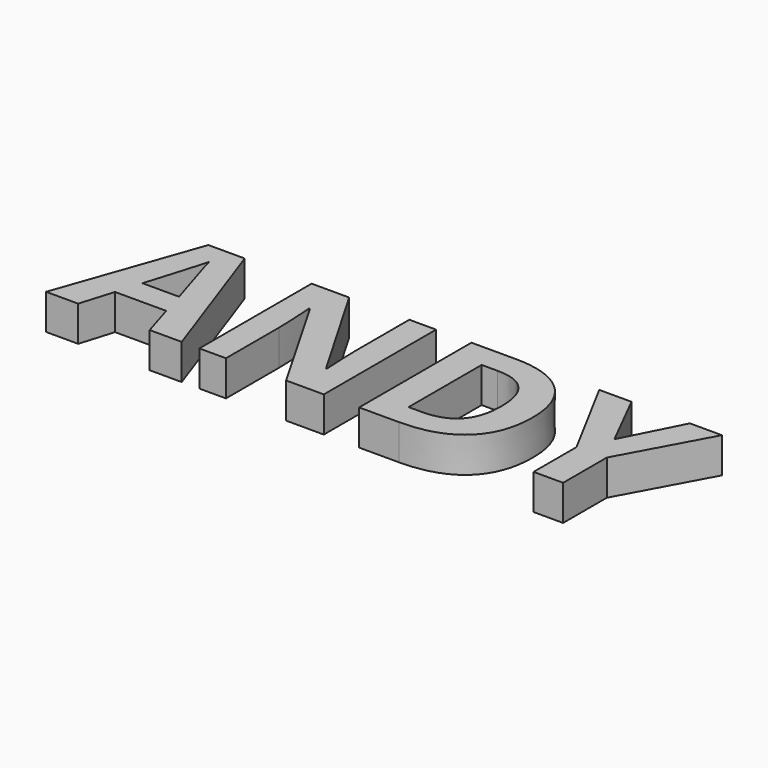
from build123d import *

# Parameters (mm, degrees)
F0_TEXT_SIZE = 11.1111111111
F1_DEPTH     = 2


# Not quite as in the source:
# - Text() gives the source's letters only with a copy of the font that has no kerning and outlines rounded to 1/6400 em; it was checked with that copy


with BuildPart() as f1:
    # F0 (on Top) → F1 (new body)
    with BuildSketch(Plane.XY):
        with Locations((7.4355997384, 8.7883091247)):
            Text('ANDY', F0_TEXT_SIZE, font='Open Sans', font_style=FontStyle.BOLD, text_align=(TextAlign.LEFT, TextAlign.BOTTOM))
    extrude(amount=F1_DEPTH)


solid = f1.part
